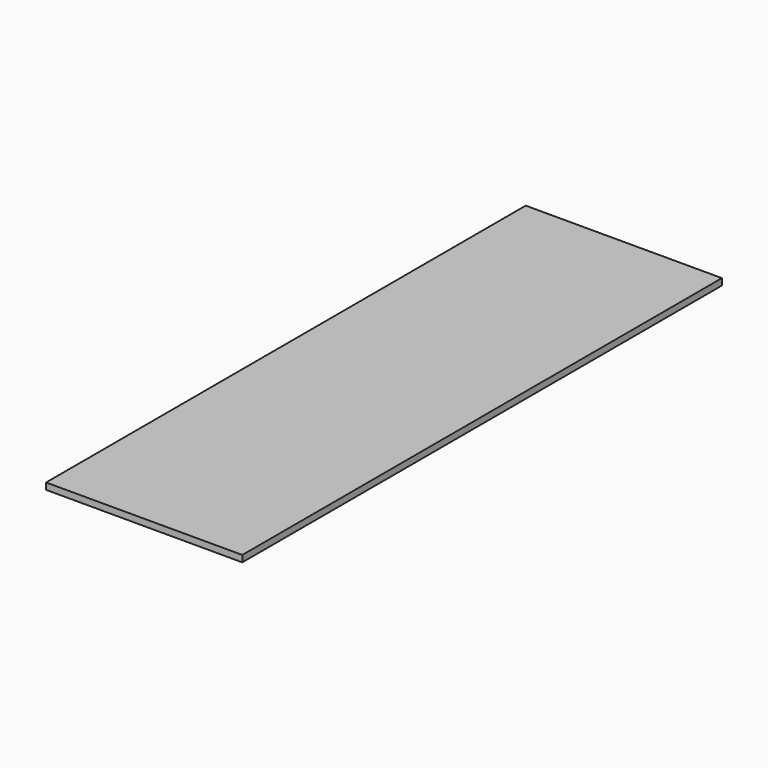
from build123d import *

# Parameters (mm, degrees)
F8_E5_RIGHT_W = 3
F8_E5_RIGHT_H = 90
F9_DEPTH      = 68
F10_DEPTH     = 207


# Not quite as in the source:
# - the program builds the solid bodies; features that only make, move or delete a surface that nothing else refers to are left out


with BuildPart() as f9:
    # F8_E5_right (on explicit) → F9 (new body)
    with BuildSketch(Plane(origin=(-50, -1.5, 26.5), x_dir=(0, 0, -1), z_dir=(0, 1, 0))):
        with Locations((1.5, 45)):
            Rectangle(F8_E5_RIGHT_W, F8_E5_RIGHT_H)
    extrude(amount=F9_DEPTH)

    # F8_E5_right (on explicit) → F10 (join)
    with BuildSketch(Plane(origin=(-50, -1.5, 26.5), x_dir=(0, 0, -1), z_dir=(0, 1, 0))):
        with Locations((1.5, 45)):
            Rectangle(F8_E5_RIGHT_W, F8_E5_RIGHT_H)
    extrude(amount=-F10_DEPTH)


solid = f9.part
